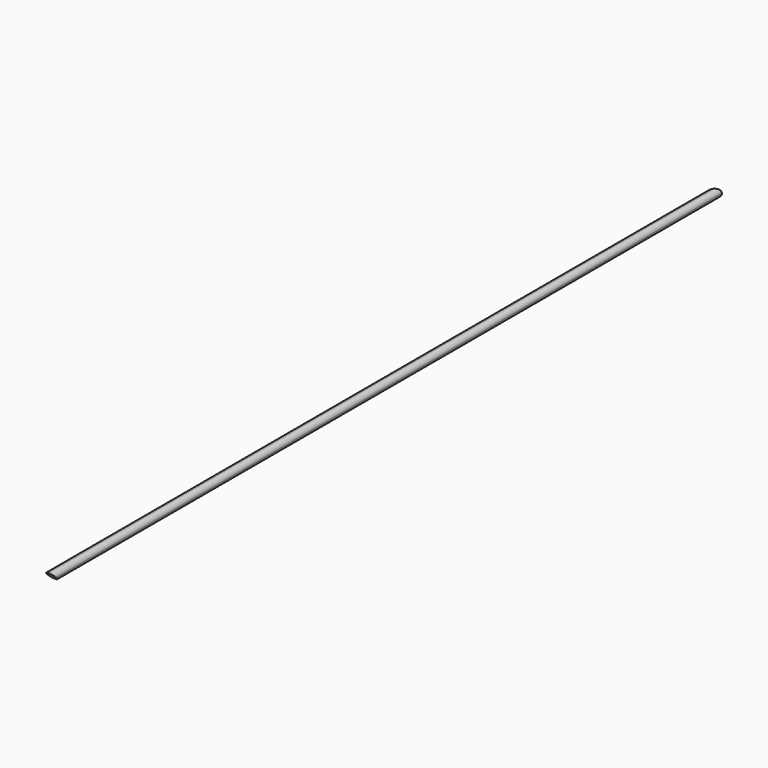
from build123d import *

# Parameters (mm, degrees)
F0_W     = 42
F0_H     = 42
F1_DEPTH = 3991
F3_DEPTH = 100
F5_DEPTH = 100
F6_R     = 20.99999


# Not quite as in the source:
# - a fillet or chamfer is up to 0.001 mm smaller than in the source, because OpenCascade refuses the exact size


with BuildPart() as f1:
    # F0 (on Front) → F1 (new body)
    with BuildSketch(Plane.XZ):
        Rectangle(F0_W, F0_H)
    extrude(amount=F1_DEPTH)

    # F2 (on face) → F3 (cut)
    with BuildSketch(Plane.YZ.offset(21)):
        Polygon((-3949, -21), (-3991, 21), (-3991, -21), align=None)
    extrude(amount=-F3_DEPTH, mode=Mode.SUBTRACT)

    # F4 (on face) → F5 (cut)
    with BuildSketch(Plane(origin=(0, 0, -21), x_dir=(1, 0, 0), z_dir=(0, 0, -1))):
        Polygon((-21, 0), (21, 0), (-21, 42), align=None)
    extrude(amount=-F5_DEPTH, mode=Mode.SUBTRACT)

    # F6 (radius 21 in the source; OpenCascade refuses exactly that, so slightly less here)
    f6_edges = [f1.edges().sort_by_distance(p)[0] for p in [
        (-21, -1995.5, -21),
        (21, -1974.5, -21),
        (21, -1995.5, 21),
        (-21, -2016.5, 21),
    ]]
    fillet(f6_edges, radius=F6_R)


solid = f1.part
